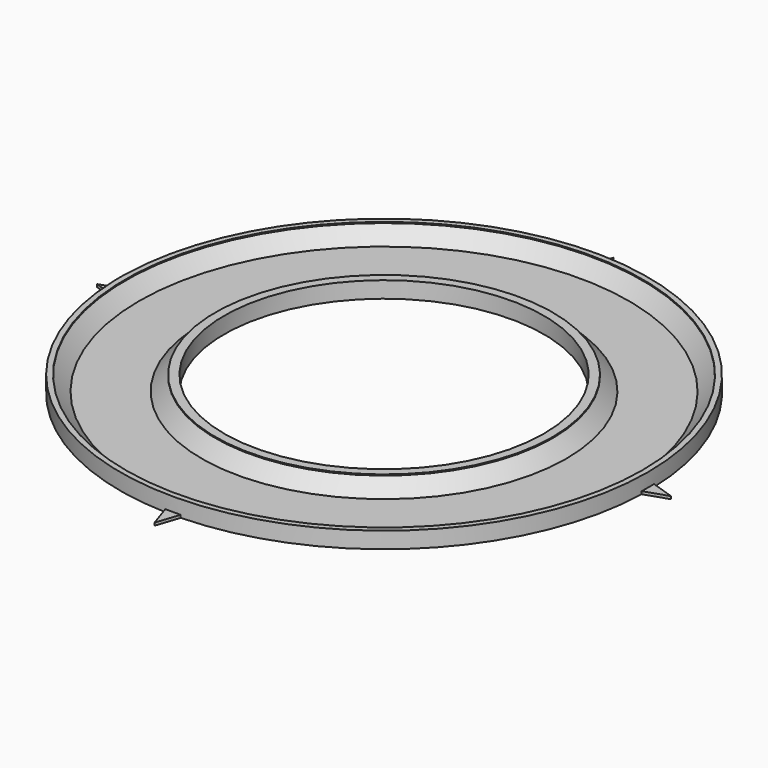
from build123d import *

# Parameters (mm, degrees)
F0_R            = 95
F0_R_2          = 62
F0_R_3          = 58.75
F1_DEPTH        = 0.6
F2_DEPTH        = 6
F3_DEPTH        = 1
F3_COPIES_COUNT = 4
F4_SIZE         = 5


# Not quite as in the source:
# - a pattern or mirror of a feature is missing from the dataset's text; its kind, count and spacing are read off the source's solid


with BuildPart() as f1:
    # F0 (on Top) → F1 (new body)
    with BuildSketch(Plane.XY):
        with BuildLine():
            ThreePointArc((-96.9585308057, -2.8360719318), (1.418187549, -96.9896321473), (97, 0))
            ThreePointArc((97, 0), (1.418187549, 96.9896321473), (-96.9585308057, 2.8360719318))
            ThreePointArc((-96.9585308057, 2.8360719318), (-96.9896321473, 1.418187549), (-97, 0))
            ThreePointArc((-97, 0), (-96.9896321473, -1.418187549), (-96.9585308057, -2.8360719318))
        make_face()
        Circle(F0_R, mode=Mode.SUBTRACT)
        Circle(F0_R)
        Circle(F0_R_2, mode=Mode.SUBTRACT)
        Circle(F0_R_2)
        Circle(F0_R_3, mode=Mode.SUBTRACT)
    extrude(amount=F1_DEPTH)

    # F0 (on Top) → F2 (join)
    with BuildSketch(Plane.XY):
        with BuildLine():
            ThreePointArc((-96.9585308057, -2.8360719318), (1.418187549, -96.9896321473), (97, 0))
            ThreePointArc((97, 0), (1.418187549, 96.9896321473), (-96.9585308057, 2.8360719318))
            ThreePointArc((-96.9585308057, 2.8360719318), (-96.9896321473, 1.418187549), (-97, 0))
            ThreePointArc((-97, 0), (-96.9896321473, -1.418187549), (-96.9585308057, -2.8360719318))
        make_face()
        Circle(F0_R, mode=Mode.SUBTRACT)
        Circle(F0_R_2)
        Circle(F0_R_3, mode=Mode.SUBTRACT)
    extrude(amount=F2_DEPTH)

    # F0 (on Top) → F3 (join)
    with BuildSketch(Plane.XY):
        with BuildLine():
            ThreePointArc((-97, 0), (-96.9896321473, 1.418187549), (-96.9585308057, 2.8360719318))
            Line((-96.9585308057, 2.8360719318), (-105.5, 0))
            Line((-105.5, 0), (-97, 0))
        make_face()
        with BuildLine():
            Line((-105.5, 0), (-96.9585308057, -2.8360719318))
            ThreePointArc((-96.9585308057, -2.8360719318), (-96.9896321473, -1.418187549), (-97, 0))
            Line((-97, 0), (-105.5, 0))
        make_face()
    f3 = extrude(amount=F3_DEPTH)

    # F3_copies: F3 ×4 about axis
    f3_copies_axis = Axis((0, 0, 0), (0, 0, 1))
    for i in range(1, F3_COPIES_COUNT):
        add(f3.rotate(f3_copies_axis, i * 360 / F3_COPIES_COUNT))

    # F4
    f4_edges = [f1.edges().sort_by_distance(p)[0] for p in [
        (-62, 0, 0.6),
        (-95, 0, 0.6),
    ]]
    chamfer(f4_edges, length=F4_SIZE)


solid = f1.part
